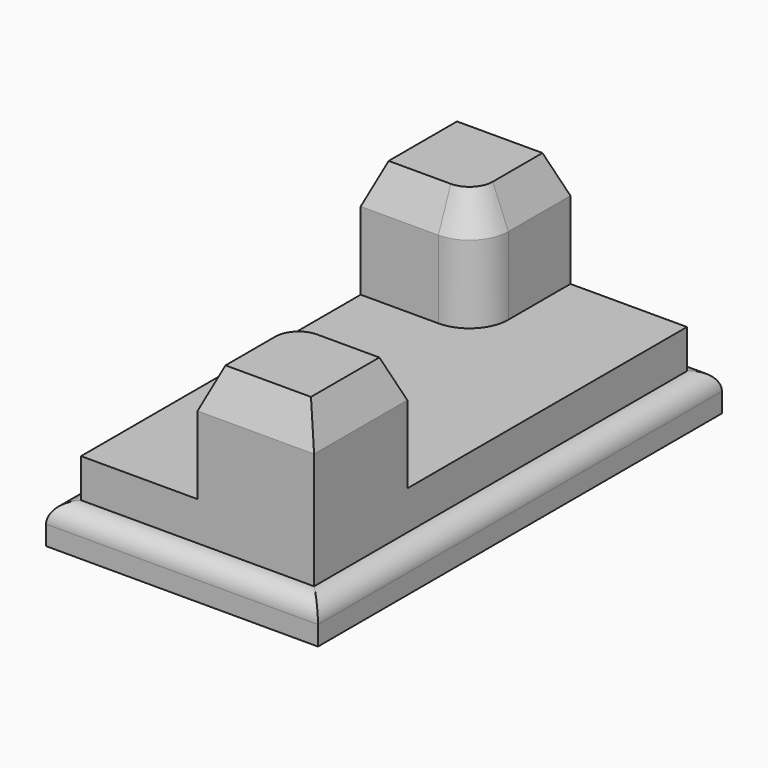
from build123d import *

# Parameters (mm, degrees)
F1_DEPTH     = 12.7
F2_DEPTH     = 25.4
F3_DEPTH     = 63.5
F4_R         = 6.34999
F5_T1_DEPTH  = 103.9650864339
F5_T3_DEPTH  = 58.332543217
F5_T5_DEPTH  = 58.332543217
F5_T7_DEPTH  = 103.9650864339
F5_T9_DEPTH  = 103.9650864339
F5_T11_DEPTH = 103.9650864339
F5_T13_DEPTH = 58.332543217
F5_T15_DEPTH = 58.332543217
F5_T18_ANGLE = 90
F5_T20_ANGLE = 90


# Not quite as in the source:
# - a fillet or chamfer that OpenCascade refuses, or shapes differently, is made with other operations: its cross-section is extruded or revolved along the edge and cut away or added
# - a fillet or chamfer is up to 0.001 mm smaller than in the source, because OpenCascade refuses the exact size
# - a feature of the source that left no trace in its solid (it failed there, or was rolled back) is left out


with BuildPart() as f1:
    # F0 (on Top) → F1 (new body)
    with BuildSketch(Plane.XY):
        Polygon((38.0595053568, 82.2464972734), (-38.0927510742, 82.2464972734), (-44.45, 82.2464972734), (-44.45, 76.2), (-44.45, -82.8535027266), (-38.1, -82.8535027266), (44.45, -82.8535027266), (44.45, 82.2464972734), align=None)
        Polygon((-38.1, -76.5035027266), (-38.1, 0), (-38.1, 37.7964972734), (-38.1, 75.8964972734), (0, 75.8964972734), (38.1, 75.8964972734), (38.1, -38.4035027266), (38.1, -76.5035027266), (0, -76.5035027266), align=None, mode=Mode.SUBTRACT)
        with BuildLine():
            Line((-38.1, 75.8964972734), (-38.1, 37.7964972734))
            Line((-38.1, 37.7964972734), (-12.7, 37.7964972734))
            ThreePointArc((-12.7, 37.7964972734), (-3.7197438789, 41.5162411524), (0, 50.4964972734))
            Line((0, 50.4964972734), (0, 75.8964972734))
            Line((0, 75.8964972734), (-38.1, 75.8964972734))
        make_face()
        with BuildLine():
            Line((-38.1, 37.7964972734), (-38.1, 0))
            Line((-38.1, 0), (-38.1, -76.5035027266))
            Line((-38.1, -76.5035027266), (0, -76.5035027266))
            Line((0, -76.5035027266), (0, -51.1035027266))
            ThreePointArc((0, -51.1035027266), (3.7197438789, -42.1232466055), (12.7, -38.4035027266))
            Line((12.7, -38.4035027266), (38.1, -38.4035027266))
            Line((38.1, -38.4035027266), (38.1, 75.8964972734))
            Line((38.1, 75.8964972734), (0, 75.8964972734))
            Line((0, 75.8964972734), (0, 50.4964972734))
            ThreePointArc((0, 50.4964972734), (-3.7197438789, 41.5162411524), (-12.7, 37.7964972734))
            Line((-12.7, 37.7964972734), (-38.1, 37.7964972734))
        make_face()
        with BuildLine():
            Line((0, -51.1035027266), (0, -76.5035027266))
            Line((0, -76.5035027266), (38.1, -76.5035027266))
            Line((38.1, -76.5035027266), (38.1, -38.4035027266))
            Line((38.1, -38.4035027266), (12.7, -38.4035027266))
            ThreePointArc((12.7, -38.4035027266), (3.7197438789, -42.1232466055), (0, -51.1035027266))
        make_face()
    extrude(amount=F1_DEPTH)

    # F0 (on Top) → F2 (join)
    with BuildSketch(Plane.XY):
        with BuildLine():
            Line((0, -51.1035027266), (0, -76.5035027266))
            Line((0, -76.5035027266), (38.1, -76.5035027266))
            Line((38.1, -76.5035027266), (38.1, -38.4035027266))
            Line((38.1, -38.4035027266), (12.7, -38.4035027266))
            ThreePointArc((12.7, -38.4035027266), (3.7197438789, -42.1232466055), (0, -51.1035027266))
        make_face()
        with BuildLine():
            Line((-38.1, 37.7964972734), (-38.1, 0))
            Line((-38.1, 0), (-38.1, -76.5035027266))
            Line((-38.1, -76.5035027266), (0, -76.5035027266))
            Line((0, -76.5035027266), (0, -51.1035027266))
            ThreePointArc((0, -51.1035027266), (3.7197438789, -42.1232466055), (12.7, -38.4035027266))
            Line((12.7, -38.4035027266), (38.1, -38.4035027266))
            Line((38.1, -38.4035027266), (38.1, 75.8964972734))
            Line((38.1, 75.8964972734), (0, 75.8964972734))
            Line((0, 75.8964972734), (0, 50.4964972734))
            ThreePointArc((0, 50.4964972734), (-3.7197438789, 41.5162411524), (-12.7, 37.7964972734))
            Line((-12.7, 37.7964972734), (-38.1, 37.7964972734))
        make_face()
        with BuildLine():
            Line((-38.1, 75.8964972734), (-38.1, 37.7964972734))
            Line((-38.1, 37.7964972734), (-12.7, 37.7964972734))
            ThreePointArc((-12.7, 37.7964972734), (-3.7197438789, 41.5162411524), (0, 50.4964972734))
            Line((0, 50.4964972734), (0, 75.8964972734))
            Line((0, 75.8964972734), (-38.1, 75.8964972734))
        make_face()
    extrude(amount=F2_DEPTH)

    # F0 (on Top) → F3 (join)
    with BuildSketch(Plane.XY):
        with BuildLine():
            Line((0, -51.1035027266), (0, -76.5035027266))
            Line((0, -76.5035027266), (38.1, -76.5035027266))
            Line((38.1, -76.5035027266), (38.1, -38.4035027266))
            Line((38.1, -38.4035027266), (12.7, -38.4035027266))
            ThreePointArc((12.7, -38.4035027266), (3.7197438789, -42.1232466055), (0, -51.1035027266))
        make_face()
        with BuildLine():
            Line((-38.1, 75.8964972734), (-38.1, 37.7964972734))
            Line((-38.1, 37.7964972734), (-12.7, 37.7964972734))
            ThreePointArc((-12.7, 37.7964972734), (-3.7197438789, 41.5162411524), (0, 50.4964972734))
            Line((0, 50.4964972734), (0, 75.8964972734))
            Line((0, 75.8964972734), (-38.1, 75.8964972734))
        make_face()
    extrude(amount=F3_DEPTH)

    # F4 (radius 6.35 in the source; OpenCascade refuses exactly that, so slightly less here)
    f4_edges = [f1.edges().sort_by_distance(p)[0] for p in [
        (-44.45, -0.303503, 12.7),
        (0, -82.853503, 12.7),
        (44.45, -0.303503, 12.7),
        (0, 82.246497, 12.7),
    ]]
    fillet(f4_edges, radius=F4_R)

    # F5: chamfer of 5.08 x 12.7 on 10 edges, made by hand

    # F5_s2 → F5_t1 (cut)
    with BuildSketch(Plane.XZ.offset(5.4709595096)):
        Polygon((38.1, 50.8), (33.02, 63.5), (38.1, 63.5), align=None)
    extrude(amount=F5_T1_DEPTH, mode=Mode.SUBTRACT)

    # F5_s4 → F5_t3 (cut)
    with BuildSketch(Plane.YZ.offset(12.7)):
        Polygon((-43.4835027266, 63.5), (-38.4035027266, 50.8), (-38.4035027266, 63.5), align=None)
    extrude(amount=F5_T3_DEPTH, mode=Mode.SUBTRACT)

    # F5_s6 → F5_t5 (cut)
    with BuildSketch(Plane.XZ.offset(51.1035027266)):
        Polygon((5.08, 63.5), (0, 50.8), (0, 63.5), align=None)
    extrude(amount=F5_T5_DEPTH, mode=Mode.SUBTRACT)

    # F5_s8 → F5_t7 (cut)
    with BuildSketch(Plane.YZ.offset(-32.932543217)):
        Polygon((-76.5035027266, 50.8), (-71.4235027266, 63.5), (-76.5035027266, 63.5), align=None)
    extrude(amount=F5_T7_DEPTH, mode=Mode.SUBTRACT)

    # F5_s10 → F5_t9 (cut)
    with BuildSketch(Plane.YZ.offset(-71.032543217)):
        Polygon((75.8964972734, 50.8), (70.8164972734, 63.5), (75.8964972734, 63.5), align=None)
    extrude(amount=F5_T9_DEPTH, mode=Mode.SUBTRACT)

    # F5_s12 → F5_t11 (cut)
    with BuildSketch(Plane.XZ.offset(-108.8290404904)):
        Polygon((-38.1, 50.8), (-33.02, 63.5), (-38.1, 63.5), align=None)
    extrude(amount=F5_T11_DEPTH, mode=Mode.SUBTRACT)

    # F5_s14 → F5_t13 (cut)
    with BuildSketch(Plane.XZ.offset(-108.8290404904)):
        Polygon((0, 50.8), (-5.08, 63.5), (0, 63.5), align=None)
    extrude(amount=F5_T13_DEPTH, mode=Mode.SUBTRACT)

    # F5_s16 → F5_t15 (cut)
    with BuildSketch(Plane.YZ.offset(-71.032543217)):
        Polygon((42.8764972734, 63.5), (37.7964972734, 50.8), (37.7964972734, 63.5), align=None)
    extrude(amount=F5_T15_DEPTH, mode=Mode.SUBTRACT)

    # F5_s17 → F5_t18 (revolve, cut)
    with BuildSketch(Plane.YZ.offset(12.7)):
        Polygon((-43.4835027266, 63.5), (-38.4035027266, 50.8), (-38.4035027266, 63.5), align=None)
    revolve(axis=Axis((12.7, -51.1035027266, 63.5), (0, 0, 1)), revolution_arc=F5_T18_ANGLE, mode=Mode.SUBTRACT)

    # F5_s19 → F5_t20 (revolve, cut)
    with BuildSketch(Plane.YZ.offset(-12.7)):
        Polygon((42.8764972734, 63.5), (37.7964972734, 50.8), (37.7964972734, 63.5), align=None)
    revolve(axis=Axis((-12.7, 50.4964972734, 63.5), (0, 0, 1)), revolution_arc=F5_T20_ANGLE, mode=Mode.SUBTRACT)


solid = f1.part
